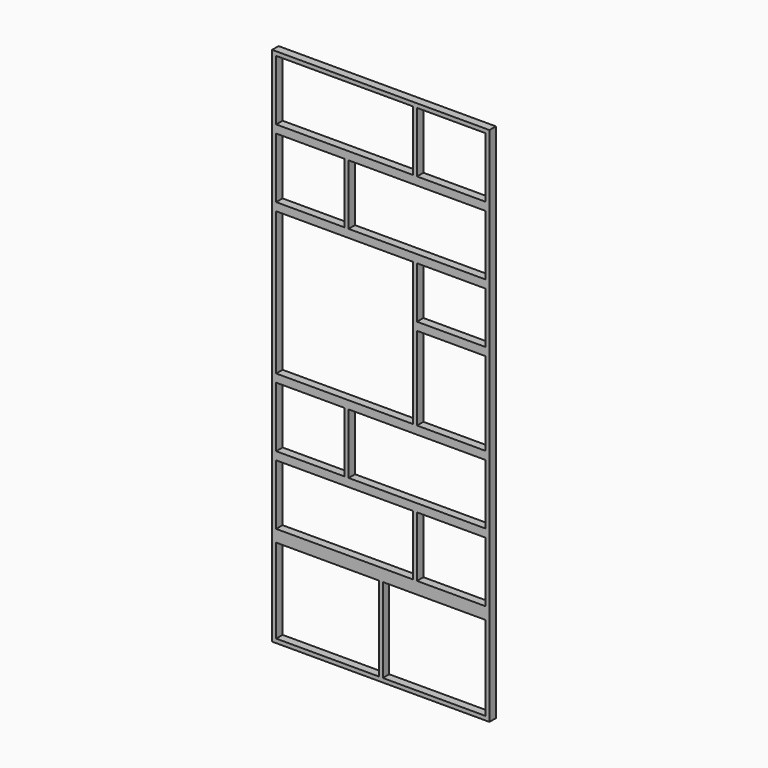
from build123d import *

# Parameters (mm, degrees)
F0_W     = 1080
F0_H     = 2590
F0_W_2   = 20
F0_H_2   = 300
F0_W_3   = 340
F0_H_3   = 40
F0_H_4   = 420
F1_DEPTH = 40


# Not quite as in the source:
# - a feature names something its author has since deleted; it is built from what else it names


with BuildPart() as f1:
    # F0 (on Front) → F1 (new body)
    with BuildSketch(Plane.XZ):
        Rectangle(F0_W, F0_H)
        Polygon((520, -855), (520, -1275), (10, -1275), (-10, -1275), (-520, -1275), (-520, -855), (-520, -795), (-520, -495), (-520, -455), (-520, -155), (-520, -115), (-520, 595), (-520, 635), (-520, 935), (-520, 975), (-520, 1275), (160, 1275), (180, 1275), (520, 1275), (520, 975), (520, 935), (520, 635), (520, 595), (520, 339.328327179), (520, 299.328327179), (520, -115), (520, -155), (520, -455), (520, -495), (520, -795), align=None, mode=Mode.SUBTRACT)
        with Locations((170, 1125)):
            Rectangle(F0_W_2, F0_H_2)
        Polygon((-160, 935), (520, 935), (520, 975), (180, 975), (160, 975), (-520, 975), (-520, 935), (-180, 935), align=None)
        with Locations((-170, 785)):
            Rectangle(F0_W_2, F0_H_2)
        Polygon((180, 595), (520, 595), (520, 635), (-160, 635), (-180, 635), (-520, 635), (-520, 595), (160, 595), align=None)
        Polygon((160, -115), (180, -115), (180, 299.328327179), (180, 339.328327179), (180, 595), (160, 595), (160, 80), (160, 40), align=None)
        with Locations((350, 319.328327179)):
            Rectangle(F0_W_3, F0_H_3)
        Polygon((-160, -155), (520, -155), (520, -115), (180, -115), (160, -115), (-520, -115), (-520, -155), (-180, -155), align=None)
        with Locations((-170, -305)):
            Rectangle(F0_W_2, F0_H_2)
        Polygon((180, -495), (520, -495), (520, -455), (-160, -455), (-180, -455), (-520, -455), (-520, -495), (160, -495), align=None)
        with Locations((170, -645)):
            Rectangle(F0_W_2, F0_H_2)
        Polygon((10, -855), (520, -855), (520, -795), (180, -795), (160, -795), (-520, -795), (-520, -855), (-10, -855), align=None)
        with Locations((0, -1065)):
            Rectangle(F0_W_2, F0_H_4)
    extrude(amount=F1_DEPTH)


solid = f1.part
